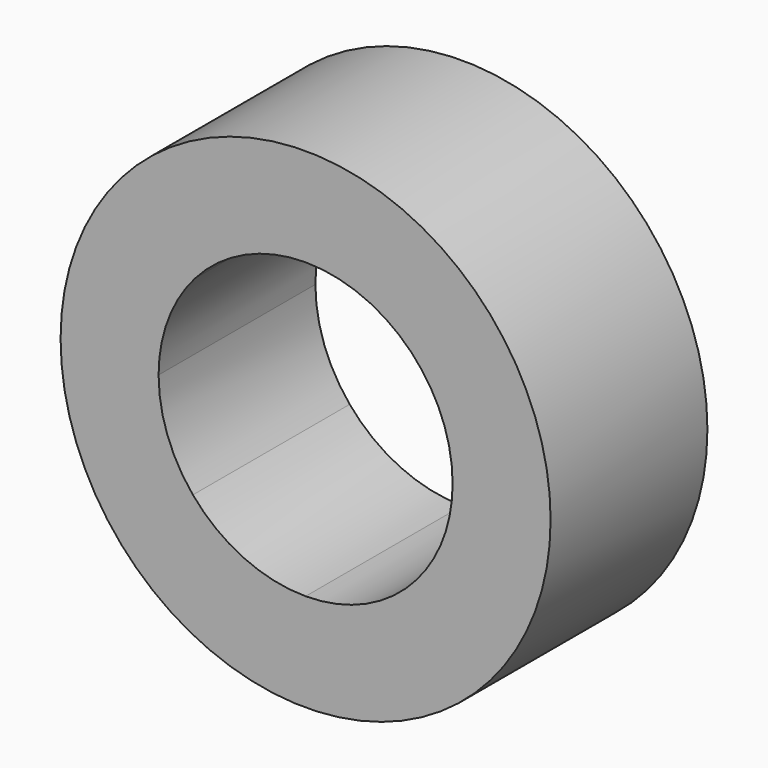
from build123d import *

# Parameters (mm, degrees)
F0_R     = 0.635
F1_DEPTH = 0.0762
F2_R     = 31.75
F4_DEPTH = 25.4
F5_DEPTH = 25.4
F6_DEPTH = 25.4


# Not quite as in the source:
# - a feature of the source that left no trace in its solid (it failed there, or was rolled back) is left out


with BuildPart() as f1:
    # F0 (on Front) → F1 (new body)
    with BuildSketch(Plane.XZ):
        Circle(F0_R)
        with BuildLine():
            ThreePointArc((0, 0.2700978897), (0.1909880494, 0.1909880494), (0.2700978897, 0))
            ThreePointArc((0.2700978897, 0), (0.1909880494, -0.1909880494), (0, -0.2700978897))
            ThreePointArc((0, -0.2700978897), (-0.1909880494, -0.1909880494), (-0.2700978897, 0))
            ThreePointArc((-0.2700978897, 0), (-0.1909880494, 0.1909880494), (0, 0.2700978897))
        make_face(mode=Mode.SUBTRACT)
    extrude(amount=F1_DEPTH)


with BuildPart() as f4:
    # F2 (on Front) → F4 (new body)
    with BuildSketch(Plane.XZ):
        Circle(F2_R)
        with BuildLine():
            ThreePointArc((13.6830996254, 13.2542553409), (17.6573716598, 7.1498060161), (19.05, 0))
            ThreePointArc((19.05, 0), (17.8415186316, -6.6770287492), (14.3694002186, -12.5069115835))
            ThreePointArc((14.3694002186, -12.5069115835), (7.8944865043, -17.3372311178), (0, -19.05))
            ThreePointArc((0, -19.05), (-8.0582243019, -17.2617357499), (-14.6035630984, -12.2326793807))
            ThreePointArc((-14.6035630984, -12.2326793807), (-17.903915452, -6.5078653557), (-19.05, 0))
            ThreePointArc((-19.05, 0), (-17.8384881524, 6.6851208244), (-14.358048248, 12.5199421128))
            ThreePointArc((-14.358048248, 12.5199421128), (-7.8866216706, 17.3408102067), (0, 19.05))
            ThreePointArc((0, 19.05), (7.4299709204, 17.5413235567), (13.6830996254, 13.2542553409))
        make_face(mode=Mode.SUBTRACT)
    extrude(amount=F4_DEPTH)

    # F2 (on Front) → F5 (join)
    with BuildSketch(Plane.XZ):
        Circle(F2_R)
        with BuildLine():
            ThreePointArc((13.6830996254, 13.2542553409), (17.6573716598, 7.1498060161), (19.05, 0))
            ThreePointArc((19.05, 0), (17.8415186316, -6.6770287492), (14.3694002186, -12.5069115835))
            ThreePointArc((14.3694002186, -12.5069115835), (7.8944865043, -17.3372311178), (0, -19.05))
            ThreePointArc((0, -19.05), (-8.0582243019, -17.2617357499), (-14.6035630984, -12.2326793807))
            ThreePointArc((-14.6035630984, -12.2326793807), (-17.903915452, -6.5078653557), (-19.05, 0))
            ThreePointArc((-19.05, 0), (-17.8384881524, 6.6851208244), (-14.358048248, 12.5199421128))
            ThreePointArc((-14.358048248, 12.5199421128), (-7.8866216706, 17.3408102067), (0, 19.05))
            ThreePointArc((0, 19.05), (7.4299709204, 17.5413235567), (13.6830996254, 13.2542553409))
        make_face(mode=Mode.SUBTRACT)
    extrude(amount=F5_DEPTH)

    # F2 (on Front) → F6 (join)
    with BuildSketch(Plane.XZ):
        Circle(F2_R)
        with BuildLine():
            ThreePointArc((13.6830996254, 13.2542553409), (17.6573716598, 7.1498060161), (19.05, 0))
            ThreePointArc((19.05, 0), (17.8415186316, -6.6770287492), (14.3694002186, -12.5069115835))
            ThreePointArc((14.3694002186, -12.5069115835), (7.8944865043, -17.3372311178), (0, -19.05))
            ThreePointArc((0, -19.05), (-8.0582243019, -17.2617357499), (-14.6035630984, -12.2326793807))
            ThreePointArc((-14.6035630984, -12.2326793807), (-17.903915452, -6.5078653557), (-19.05, 0))
            ThreePointArc((-19.05, 0), (-17.8384881524, 6.6851208244), (-14.358048248, 12.5199421128))
            ThreePointArc((-14.358048248, 12.5199421128), (-7.8866216706, 17.3408102067), (0, 19.05))
            ThreePointArc((0, 19.05), (7.4299709204, 17.5413235567), (13.6830996254, 13.2542553409))
        make_face(mode=Mode.SUBTRACT)
    extrude(amount=F6_DEPTH)


solid = Compound([f1.part, f4.part])
